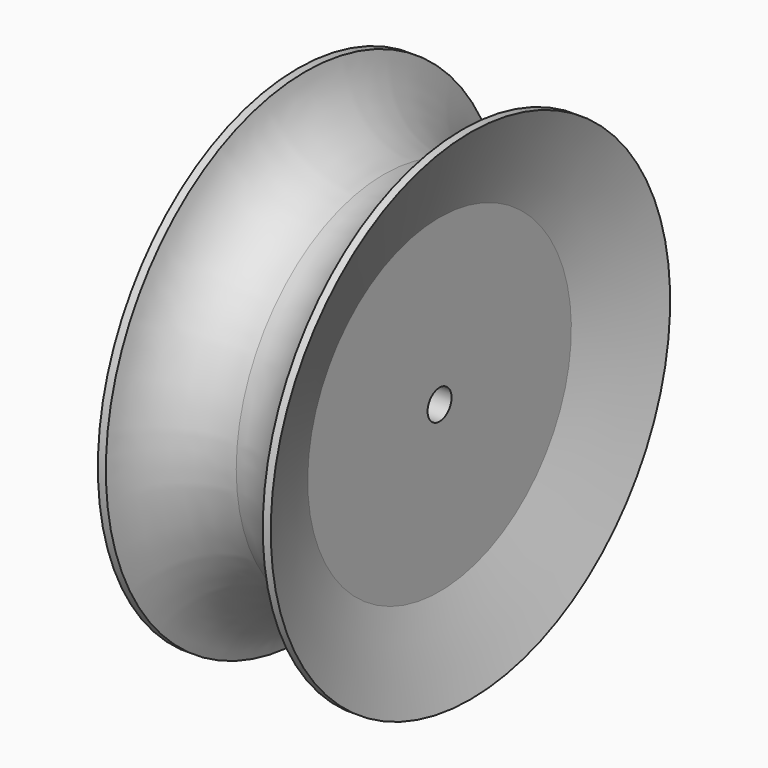
from build123d import *
from build123d import SkipClean  # not in build123d's __all__


with BuildPart() as f1:
    # F0 (on Front) → F1 (revolve)
    with BuildSketch(Plane.XZ):
        with BuildLine():
            Line((0, 15), (55.6436983149, 15))
            Line((55.6436983149, 15), (55.6436983149, 165))
            Line((55.6436983149, 165), (86.5811682275, 250))
            Line((86.5811682275, 250), (78.5811682275, 250))
            ThreePointArc((78.5811682275, 250), (50.9901951359, 203.3558599703), (0, 185))
            Line((0, 185), (0, 15))
        make_face()
    revolve(axis=Axis((-5.425222218, 0, 0), (1, 0, 0)))

    # F2: F1 across plane


with BuildPart() as f1_1:
    add(f1.part, clean=False)
    with SkipClean():  # cleaning this boolean's faces spoils the solid; the shape is the same uncleaned
        add(f1.part.mirror(Plane.YZ), clean=False)


solid = f1_1.part
